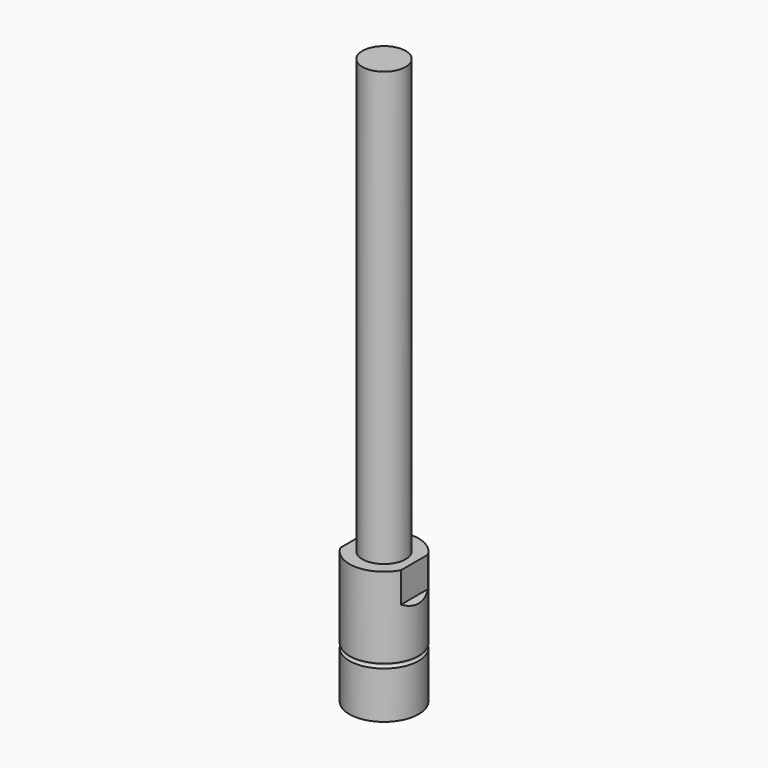
from build123d import *

# Parameters (mm, degrees)
F2_W     = 19.6017324924
F2_H     = 37.1457748115
F2_W_2   = 14
F2_H_2   = 30
F3_DEPTH = 8
F4_SIZE  = 0.99999


# Not quite as in the source:
# - a fillet or chamfer is up to 0.001 mm smaller than in the source, because OpenCascade refuses the exact size


with BuildPart() as f1:
    # F0 (on Front) → F1 (revolve)
    with BuildSketch(Plane.XZ):
        with BuildLine():
            Line((2.9315422289, 21.0469197482), (2.9315422289, 0))
            Line((2.9315422289, 0), (8, 0))
            Line((8, 0), (8, 10.8380244002))
            ThreePointArc((8, 10.8380244002), (7.5, 11.3380244002), (8, 11.8380244002))
            Line((8, 11.8380244002), (8, 30.5))
            Line((8, 30.5), (5, 30.5))
            Line((5, 30.5), (5, 130.5))
            Line((5, 130.5), (0, 130.5))
            Line((0, 130.5), (0, 30.5))
            Line((0, 30.5), (0, 21.0469197482))
            Line((0, 21.0469197482), (2.9315422289, 21.0469197482))
        make_face()
    revolve(axis=Axis((0, 0, 80.5), (0, 0, 1)))

    # F2 (on face) → F3 (cut)
    with BuildSketch(Plane.XY.offset(30.5)):
        Rectangle(F2_W, F2_H)
        Rectangle(F2_W_2, F2_H_2, mode=Mode.SUBTRACT)
    extrude(amount=-F3_DEPTH, mode=Mode.SUBTRACT)

    # F4 (size 1 in the source; OpenCascade refuses exactly that, so slightly less here)
    f4_edges = [f1.edges().sort_by_distance(p)[0] for p in [
        (-7, 0, 22.5),
        (7, 0, 22.5),
    ]]
    chamfer(f4_edges, length=F4_SIZE)


solid = f1.part
